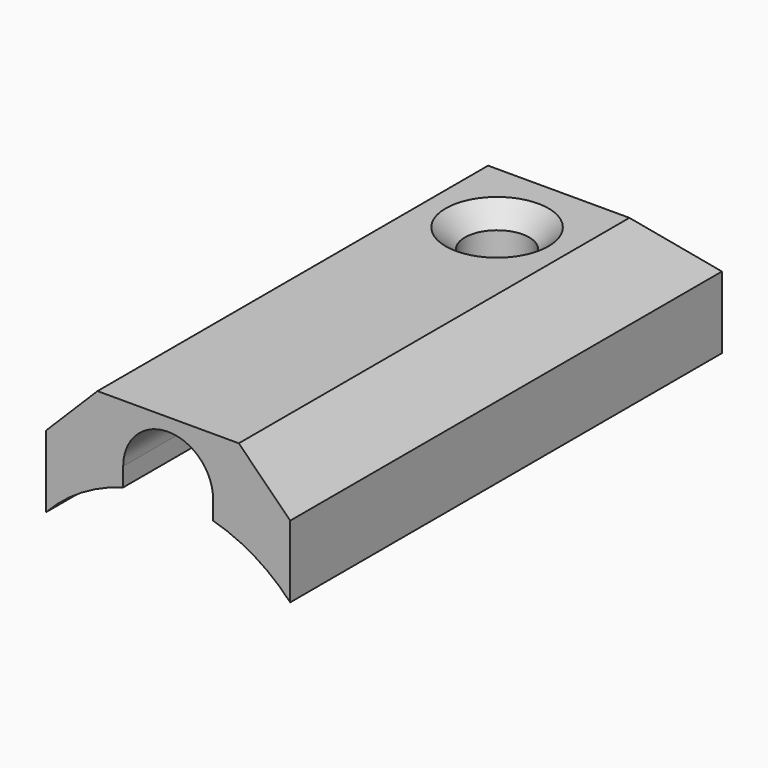
from build123d import *

# Parameters (mm, degrees)
F6_DEPTH        = 21
F7_SIZE         = 2
F8_SIZE         = 2
F12_DEPTH       = 2.5510001
F14_D           = 2.5
F14_CSINK_D     = 4
F14_CSINK_ANGLE = 90


# Not quite as in the source:
# - a feature names something its author has since deleted; it is built from what else it names


with BuildPart() as f6:
    # F5 (on Front) → F6 (new body)
    with BuildSketch(Plane.XZ):
        with BuildLine():
            ThreePointArc((1.75, 6.2599920128), (3.3753918927, 5.5548833985), (4.75, 4.4370598373))
            Line((4.75, 4.4370598373), (4.75, 9.2370598373))
            Line((4.75, 9.2370598373), (-4.75, 9.2370598373))
            Line((-4.75, 9.2370598373), (-4.75, 4.4370598373))
            ThreePointArc((-4.75, 4.4370598373), (-3.3753918927, 5.5548833985), (-1.75, 6.2599920128))
            Line((-1.75, 6.2599920128), (-1.75, 6.9870598373))
            ThreePointArc((-1.75, 6.9870598373), (0, 8.7370598373), (1.75, 6.9870598373))
            Line((1.75, 6.9870598373), (1.75, 6.2599920128))
        make_face()
        with BuildLine():
            ThreePointArc((-1.75, 6.2599920128), (0, 6.5), (1.75, 6.2599920128))
            Line((1.75, 6.2599920128), (1.75, 6.9870598373))
            ThreePointArc((1.75, 6.9870598373), (0, 8.7370598373), (-1.75, 6.9870598373))
            Line((-1.75, 6.9870598373), (-1.75, 6.2599920128))
        make_face()
    extrude(amount=-F6_DEPTH)

    # F7
    f7_edges = [f6.edges().sort_by_distance(p)[0] for p in [
        (-4.75, 10.5, 9.23706),
        (4.75, 10.5, 9.23706),
    ]]
    chamfer(f7_edges, length=F7_SIZE)

    # F8
    f8_edges = [f6.edges().sort_by_distance(p)[0] for p in [
        (0, 21, 9.23706),
    ]]
    chamfer(f8_edges, length=F8_SIZE)

    # F10 (on offset) → F11 (revolve, cut)
    with BuildSketch(Plane.XY.offset(6.9870598373)):
        with BuildLine():
            Line((-1.75, 11.75), (-1.75, 0))
            Line((-1.75, 0), (0, 0))
            Line((0, 0), (0, 13.5))
            ThreePointArc((0, 13.5), (-1.2374368671, 12.9874368671), (-1.75, 11.75))
        make_face()
    revolve(axis=Axis((0, 6.75, 6.9870598373), (0, 1, 0)), mode=Mode.SUBTRACT)

    # F10 (on offset) → F12 (cut, through all)
    with BuildSketch(Plane.XY.offset(6.9870598373)):
        with BuildLine():
            Line((0, 13.5), (0, 0))
            Line((0, 0), (1.75, 0))
            Line((1.75, 0), (1.75, 11.75))
            ThreePointArc((1.75, 11.75), (1.2374368671, 12.9874368671), (0, 13.5))
        make_face()
        with BuildLine():
            Line((-1.75, 11.75), (-1.75, 0))
            Line((-1.75, 0), (0, 0))
            Line((0, 0), (0, 13.5))
            ThreePointArc((0, 13.5), (-1.2374368671, 12.9874368671), (-1.75, 11.75))
        make_face()
    extrude(amount=-F12_DEPTH, mode=Mode.SUBTRACT)

    # F14 (through all)
    with Locations(Plane.XY.offset(9.2370598373)):
        with Locations((0, 16)):
            CounterSinkHole(F14_D / 2, F14_CSINK_D / 2, counter_sink_angle=F14_CSINK_ANGLE)


solid = f6.part
